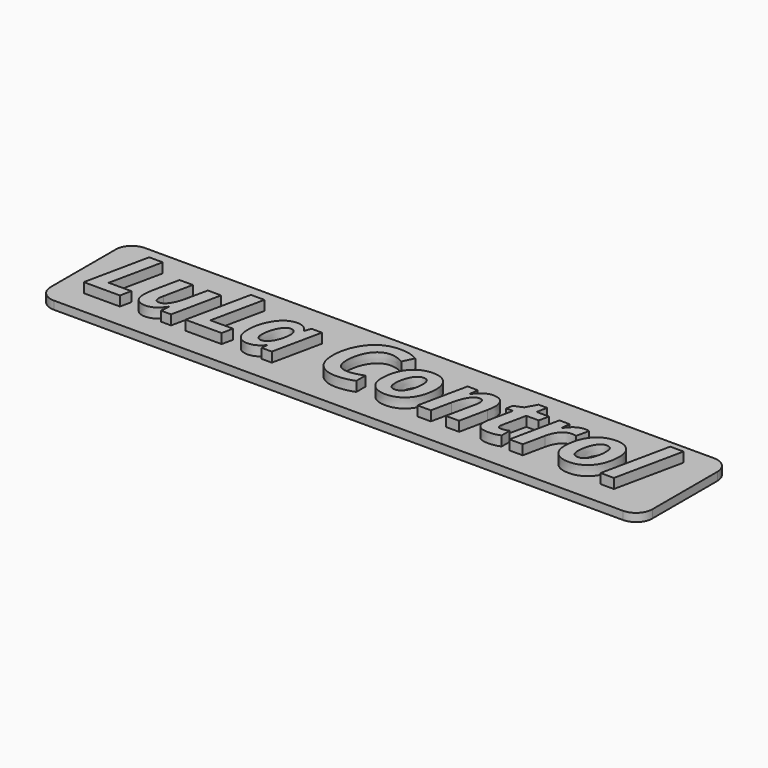
from build123d import *

# Parameters (mm, degrees)
F1_DEPTH     = 0.5
F2_TEXT_SIZE = 5.5714870955
F3_DEPTH     = 0.6


# Not quite as in the source:
# - Text() gives the source's letters only with a copy of the font that has no kerning and outlines rounded to 1/6400 em; it was checked with that copy


with BuildPart() as f1:
    # F0 (on Top) → F1 (new body)
    with BuildSketch(Plane.XY):
        with BuildLine():
            Line((17.5, 3.5), (-17.5, 3.5))
            ThreePointArc((-17.5, 3.5), (-18.2071067812, 3.2071067812), (-18.5, 2.5))
            Line((-18.5, 2.5), (-18.5, -2.5))
            ThreePointArc((-18.5, -2.5), (-18.2071067812, -3.2071067812), (-17.5, -3.5))
            Line((-17.5, -3.5), (17.5, -3.5))
            ThreePointArc((17.5, -3.5), (18.2071067812, -3.2071067812), (18.5, -2.5))
            Line((18.5, -2.5), (18.5, 2.5))
            ThreePointArc((18.5, 2.5), (18.2071067812, 3.2071067812), (17.5, 3.5))
        make_face()
    extrude(amount=F1_DEPTH)

    # F2 (on face) → F3 (join)
    with BuildSketch(Plane.XY.offset(0.5)):
        with Locations((-17, -2.0073056316)):
            Text('LuLa Control', F2_TEXT_SIZE, font='Open Sans', font_style=FontStyle.BOLDITALIC, text_align=(TextAlign.LEFT, TextAlign.BOTTOM))
    extrude(amount=F3_DEPTH)


solid = f1.part
